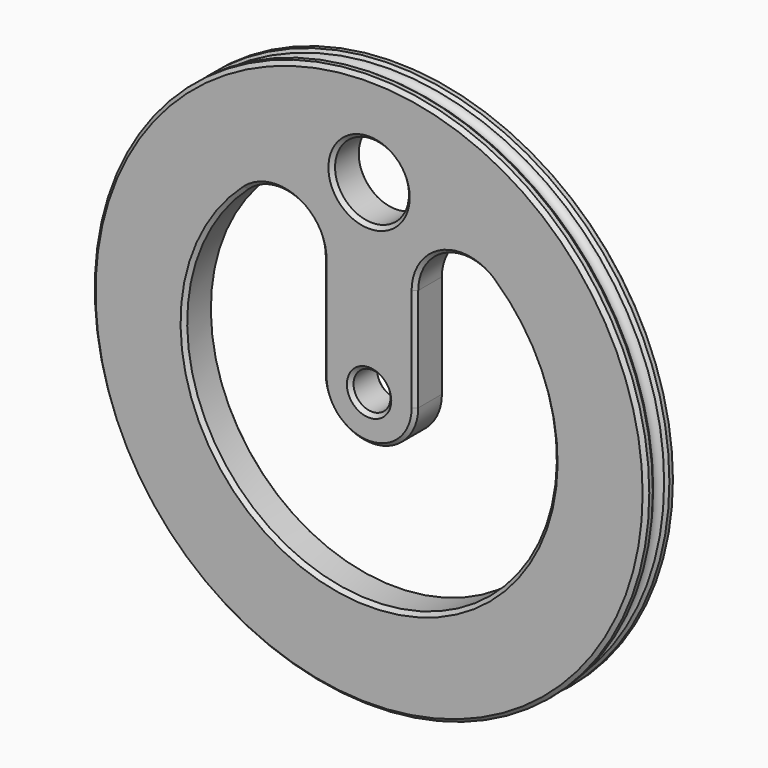
from build123d import *

# Parameters (mm, degrees)
F0_R         = 38.1
F0_R_2       = 2.54
F0_R_3       = 5.08
F1_DEPTH     = 5.08
F5_T1_DEPTH  = 14.1990316571
F5_T6_ANGLE  = 276.3793702084
F5_T8_ANGLE  = 131.8103148958
F5_T10_ANGLE = 180
F5_T12_ANGLE = 131.8103148958
F5_T20_ANGLE = 276.3793702084
F5_T22_ANGLE = 131.8103148958
F5_T24_ANGLE = 180
F5_T26_ANGLE = 131.8103148958
F5_T32_ANGLE = 270
F5_T34_ANGLE = 90
F5_T36_ANGLE = 90
F5_T38_ANGLE = 270


# Not quite as in the source:
# - a fillet or chamfer that OpenCascade refuses, or shapes differently, is made with other operations: its cross-section is extruded or revolved along the edge and cut away or added


with BuildPart() as f1:
    # F0 (on Front) → F1 (new body)
    with BuildSketch(Plane.XZ):
        Circle(F0_R)
        with BuildLine():
            ThreePointArc((16.9333333333, 18.9320422095), (0, -25.4), (-16.9333333333, 18.9320422095))
            ThreePointArc((-16.9333333333, 18.9320422095), (-10.1076233556, 19.9957620574), (-6.35, 14.1990316571))
            Line((-6.35, 14.1990316571), (-6.35, 0))
            ThreePointArc((-6.35, 0), (-4.4901280605, -4.4901280605), (0, -6.35))
            ThreePointArc((0, -6.35), (4.4901280605, -4.4901280605), (6.35, 0))
            Line((6.35, 0), (6.35, 14.1990316571))
            ThreePointArc((6.35, 14.1990316571), (10.1076233556, 19.9957620574), (16.9333333333, 18.9320422095))
        make_face(mode=Mode.SUBTRACT)
        Circle(F0_R_2, mode=Mode.SUBTRACT)
        with Locations((0, 25.4)):
            Circle(F0_R_3, mode=Mode.SUBTRACT)
    extrude(amount=F1_DEPTH)


with BuildPart() as f3:
    # F2 (on Right) → F3 (revolve)
    with BuildSketch(Plane.YZ):
        with BuildLine():
            ThreePointArc((-3.54, 38.1), (-2.54, 37.1), (-1.54, 38.1))
            Line((-1.54, 38.1), (-3.54, 38.1))
        make_face()
        with BuildLine():
            Line((-3.54, 38.1), (-1.54, 38.1))
            ThreePointArc((-1.54, 38.1), (-2.54, 39.1), (-3.54, 38.1))
        make_face()
    revolve(axis=Axis((0, 0, 0), (0, -1, 0)))


with BuildPart() as f1_1:
    add(f1.part)

    # F4: cut F3
    add(f3.part, mode=Mode.SUBTRACT)

    # F5: chamfer of 0.508 on 22 edges, made by hand

    # F5_s2 → F5_t1 (cut)
    with BuildSketch(Plane.XY):
        Polygon((-6.35, -4.572), (-5.842, -5.08), (-6.35, -5.08), align=None)
        Polygon((6.35, -4.572), (5.842, -5.08), (6.35, -5.08), align=None)
        Polygon((-5.842, 0), (-6.35, -0.508), (-6.35, 0), align=None)
        Polygon((5.842, 0), (6.35, -0.508), (6.35, 0), align=None)
    extrude(amount=F5_T1_DEPTH, mode=Mode.SUBTRACT)

    # F5_s3 → F5_t4 (revolve, cut)
    with BuildSketch(Plane.XY):
        Polygon((38.1, -4.572), (37.592, -5.08), (38.1, -5.08), align=None)
    revolve(axis=Axis((0, -5.08, 0), (0, -1, 0)), mode=Mode.SUBTRACT)

    # F5_s5 → F5_t6 (revolve, cut)
    with BuildSketch(Plane(origin=(0, 0, 0), x_dir=(0, 1, 0), z_dir=(-0.7453559925, 0, 0.6666666667))):
        Polygon((-4.572, -25.4), (-5.08, -25.908), (-5.08, -25.4), align=None)
    revolve(axis=Axis((0, -5.08, 0), (0, 1, 0)), revolution_arc=F5_T6_ANGLE, mode=Mode.SUBTRACT)

    # F5_s7 → F5_t8 (revolve, cut)
    with BuildSketch(Plane(origin=(0, 0, 0), x_dir=(0, 1, 0), z_dir=(-0.7453559925, 0, -0.6666666667))):
        Polygon((-4.572, -25.4), (-5.08, -25.908), (-5.08, -25.4), align=None)
    revolve(axis=Axis((-12.7, -5.08, 14.1990316571), (0, 1, 0)), revolution_arc=F5_T8_ANGLE, mode=Mode.SUBTRACT)

    # F5_s9 → F5_t10 (revolve, cut)
    with BuildSketch(Plane.XY):
        Polygon((6.35, -4.572), (5.842, -5.08), (6.35, -5.08), align=None)
    revolve(axis=Axis((0, -5.08, 0), (0, 1, 0)), revolution_arc=F5_T10_ANGLE, mode=Mode.SUBTRACT)

    # F5_s11 → F5_t12 (revolve, cut)
    with BuildSketch(Plane.XY.offset(14.1990316571)):
        Polygon((6.35, -4.572), (5.842, -5.08), (6.35, -5.08), align=None)
    revolve(axis=Axis((12.7, -5.08, 14.1990316571), (0, 1, 0)), revolution_arc=F5_T12_ANGLE, mode=Mode.SUBTRACT)

    # F5_s13 → F5_t14 (revolve, cut)
    with BuildSketch(Plane.XY):
        Polygon((2.54, -4.572), (3.048, -5.08), (2.54, -5.08), align=None)
    revolve(axis=Axis((0, -5.08, 0), (0, -1, 0)), mode=Mode.SUBTRACT)

    # F5_s15 → F5_t16 (revolve, cut)
    with BuildSketch(Plane.XY.offset(25.4)):
        Polygon((5.08, -4.572), (5.588, -5.08), (5.08, -5.08), align=None)
    revolve(axis=Axis((0, -5.08, 25.4), (0, -1, 0)), mode=Mode.SUBTRACT)

    # F5_s17 → F5_t18 (revolve, cut)
    with BuildSketch(Plane.XY):
        Polygon((38.1, -0.508), (37.592, 0), (38.1, 0), align=None)
    revolve(axis=Axis((0, 0, 0), (0, -1, 0)), mode=Mode.SUBTRACT)

    # F5_s19 → F5_t20 (revolve, cut)
    with BuildSketch(Plane(origin=(0, 0, 0), x_dir=(0, 1, 0), z_dir=(-0.7453559925, 0, 0.6666666667))):
        Polygon((0, -25.908), (-0.508, -25.4), (0, -25.4), align=None)
    revolve(axis=Axis((0, 0, 0), (0, 1, 0)), revolution_arc=F5_T20_ANGLE, mode=Mode.SUBTRACT)

    # F5_s21 → F5_t22 (revolve, cut)
    with BuildSketch(Plane(origin=(0, 0, 0), x_dir=(0, 1, 0), z_dir=(-0.7453559925, 0, -0.6666666667))):
        Polygon((0, -25.908), (-0.508, -25.4), (0, -25.4), align=None)
    revolve(axis=Axis((-12.7, 0, 14.1990316571), (0, 1, 0)), revolution_arc=F5_T22_ANGLE, mode=Mode.SUBTRACT)

    # F5_s23 → F5_t24 (revolve, cut)
    with BuildSketch(Plane.XY):
        Polygon((-5.842, 0), (-6.35, -0.508), (-6.35, 0), align=None)
    revolve(axis=Axis((0, 0, 0), (0, -1, 0)), revolution_arc=F5_T24_ANGLE, mode=Mode.SUBTRACT)

    # F5_s25 → F5_t26 (revolve, cut)
    with BuildSketch(Plane.XY.offset(14.1990316571)):
        Polygon((5.842, 0), (6.35, -0.508), (6.35, 0), align=None)
    revolve(axis=Axis((12.7, 0, 14.1990316571), (0, 1, 0)), revolution_arc=F5_T26_ANGLE, mode=Mode.SUBTRACT)

    # F5_s27 → F5_t28 (revolve, cut)
    with BuildSketch(Plane.XY):
        Polygon((3.048, 0), (2.54, -0.508), (2.54, 0), align=None)
    revolve(axis=Axis((0, 0, 0), (0, -1, 0)), mode=Mode.SUBTRACT)

    # F5_s29 → F5_t30 (revolve, cut)
    with BuildSketch(Plane.XY.offset(25.4)):
        Polygon((5.588, 0), (5.08, -0.508), (5.08, 0), align=None)
    revolve(axis=Axis((0, 0, 25.4), (0, -1, 0)), mode=Mode.SUBTRACT)

    # F5_s31 → F5_t32 (revolve, cut)
    with BuildSketch(Plane.YZ):
        with BuildLine():
            Line((-1.1201408521, 38.1), (-1.5984488409, 37.7631299735))
            ThreePointArc((-1.5984488409, 37.7631299735), (-1.5560027564, 37.921816318), (-1.54, 38.1))
            Line((-1.54, 38.1), (-1.1201408521, 38.1))
        make_face()
    revolve(axis=Axis((0, -1.54, 0), (0, -1, 0)), revolution_arc=F5_T32_ANGLE, mode=Mode.SUBTRACT)

    # F5_s33 → F5_t34 (revolve, cut)
    with BuildSketch(Plane.XY):
        with BuildLine():
            Line((38.1, -1.1201408521), (37.7631299735, -1.5984488409))
            ThreePointArc((37.7631299735, -1.5984488409), (37.921816318, -1.5560027564), (38.1, -1.54))
            Line((38.1, -1.54), (38.1, -1.1201408521))
        make_face()
    revolve(axis=Axis((0, -1.54, 0), (0, -1, 0)), revolution_arc=F5_T34_ANGLE, mode=Mode.SUBTRACT)

    # F5_s35 → F5_t36 (revolve, cut)
    with BuildSketch(Plane.XY):
        with BuildLine():
            Line((37.7631299735, -3.4815511591), (38.1, -3.9598591479))
            Line((38.1, -3.9598591479), (38.1, -3.54))
            ThreePointArc((38.1, -3.54), (37.921816318, -3.5239972436), (37.7631299735, -3.4815511591))
        make_face()
    revolve(axis=Axis((0, -3.54, 0), (0, -1, 0)), revolution_arc=F5_T36_ANGLE, mode=Mode.SUBTRACT)

    # F5_s37 → F5_t38 (revolve, cut)
    with BuildSketch(Plane.YZ):
        with BuildLine():
            Line((-3.4815511591, 37.7631299735), (-3.9598591479, 38.1))
            Line((-3.9598591479, 38.1), (-3.54, 38.1))
            ThreePointArc((-3.54, 38.1), (-3.5239972436, 37.921816318), (-3.4815511591, 37.7631299735))
        make_face()
    revolve(axis=Axis((0, -3.54, 0), (0, -1, 0)), revolution_arc=F5_T38_ANGLE, mode=Mode.SUBTRACT)


solid = f1_1.part
